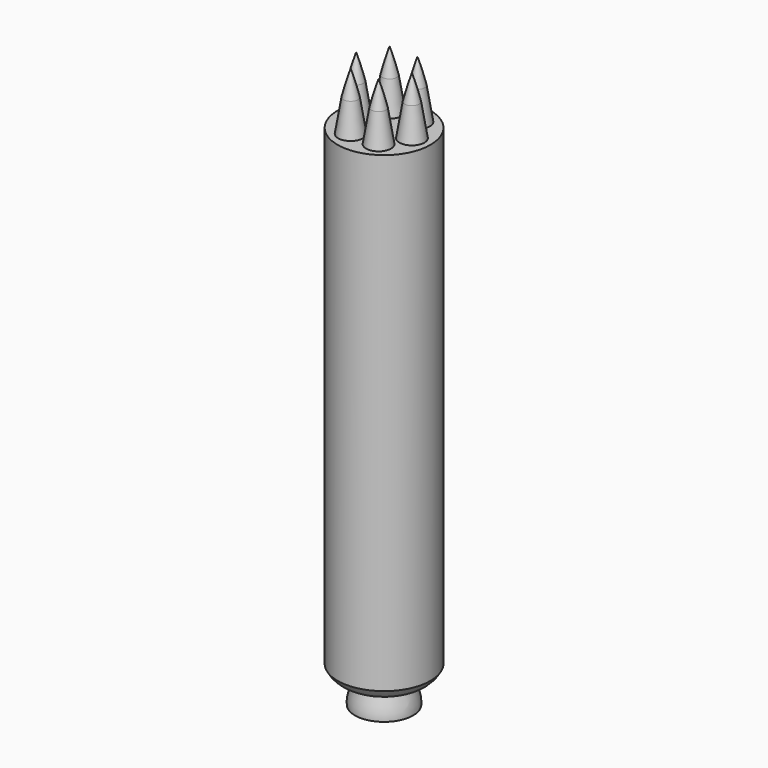
from build123d import *

# Parameters (mm, degrees)
F6_COUNT = 6


# Not quite as in the source:
# - a feature names something its author has since deleted; it is built from what else it names


with BuildPart() as f1:
    # F0 (on Front) → F1 (revolve)
    with BuildSketch(Plane.XZ):
        with BuildLine():
            Line((-6.8414350972, 19.2343222741), (-6.8414350972, -46.4227162302))
            Line((-6.8414350972, -46.4227162302), (-3.0813866761, -46.4227162302))
            add(Edge.make_bspline(
                [(-3.6481511779, -43.5762032866), (-3.395314794, -44.2455634475), (-2.95054866, -45.8208620548), (-3.0813866761, -46.4227162302)],
                knots=[0, 0, 0, 0, 2.9023883162, 2.9023883162, 2.9023883162, 2.9023883162], degree=3))
            add(Edge.make_bspline(
                [(-0.8414350972, -41.7563058436), (-1.4245474534, -42.9885461926), (-2.6062515099, -43.3626174927), (-3.6481511779, -43.5762032866)],
                knots=[0, 0, 0, 0, 3.3450981841, 3.3450981841, 3.3450981841, 3.3450981841], degree=3))
            Line((-0.8414350972, -41.7563058436), (-0.8414350972, 19.2343222741))
            Line((-0.8414350972, 19.2343222741), (-6.8414350972, 19.2343222741))
        make_face()
    revolve(axis=Axis((-6.8414350972, 0, -0.2756823954), (0, 0, 1)))


with BuildPart() as f5:
    # F4 (on face) → F5 (revolve)
    with BuildSketch(Plane(origin=(-8.863033166, -0.7754149265, 0), x_dir=(-0.0871557427, 0.9961946981, 0), z_dir=(0.9961946981, 0.0871557427, 0))):
        with BuildLine():
            Line((-3.2882800627, 23.3996900685), (-3.9674532244, 19.2343222741))
            Line((-3.9674532244, 19.2343222741), (-2.3581811491, 19.2343222741))
            Line((-2.3581811491, 19.2343222741), (-2.3581811491, 21.2729978624))
            Line((-2.3581811491, 21.2729978624), (-2.3581811491, 22.6256599784))
            Line((-2.3581811491, 22.6256599784), (-2.3581811491, 26.6642030329))
            ThreePointArc((-2.3581811491, 26.6642030329), (-2.8576228531, 25.0417453146), (-3.2882800627, 23.3996900685))
        make_face()
    revolve(axis=Axis((-8.6575041364, -3.1246224843, 20.2536600682), (0, 0, 1)))


with BuildPart() as f6_1:
    # F6: instance of F5
    add(f5.part.rotate(Axis((-6.8414350972, 0, -0.2756823954), (0, 0, 1)), 1 * 360 / F6_COUNT))


with BuildPart() as f6_2:
    # F6: instance of F5
    add(f5.part.rotate(Axis((-6.8414350972, 0, -0.2756823954), (0, 0, 1)), 2 * 360 / F6_COUNT))


with BuildPart() as f6_3:
    # F6: instance of F5
    add(f5.part.rotate(Axis((-6.8414350972, 0, -0.2756823954), (0, 0, 1)), 3 * 360 / F6_COUNT))


with BuildPart() as f6_4:
    # F6: instance of F5
    add(f5.part.rotate(Axis((-6.8414350972, 0, -0.2756823954), (0, 0, 1)), 4 * 360 / F6_COUNT))


with BuildPart() as f6_5:
    # F6: instance of F5
    add(f5.part.rotate(Axis((-6.8414350972, 0, -0.2756823954), (0, 0, 1)), 5 * 360 / F6_COUNT))


solid = Compound([f1.part, f5.part, f6_1.part, f6_2.part, f6_3.part, f6_4.part, f6_5.part])
